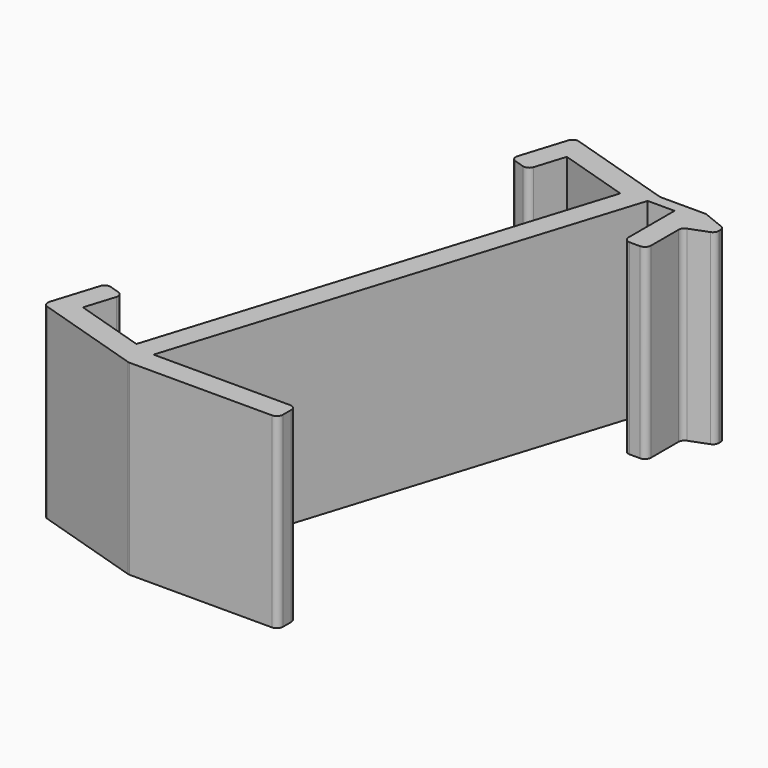
from build123d import *

# Parameters (mm, degrees)
F1_DEPTH = 25
F2_R     = 0.8


# Not quite as in the source:
# - a feature names something its author has since deleted; it is built from what else it names


with BuildPart() as f1:
    # F0 (on Top) → F1 (new body)
    with BuildSketch(Plane.XY):
        Polygon((-15.2705168036, 4.776119403), (-17.6585765051, -2.8591389988), (-14.7953546044, -3.7546613869), (-13.302817291, 1.0173751143), (-3.7587442887, -1.9676995126), (-21.9676995126, -60.1865448263), (-31.5117725148, -57.2014701994), (-30.0192352014, -52.4294336983), (-32.8824571021, -51.5339113102), (-35.2705168036, -59.169169712), (-20, -63.945289115), (-19.0616978853, -60.945289115), (-0.4691510573, -1.5), (3.1308489427, -1.5), (3.1308489427, -10), (6.1308489427, -10), (6.1308489427, -4.0311980993), (6.1308489427, 0), (0, 0), align=None)
        Polygon((0, -60.945289115), (-19.0616978853, -60.945289115), (-20, -63.945289115), (0, -63.945289115), align=None)
        Polygon((9.5918557882, -1.385692507), (6.1308489427, 0), (6.1308489427, -4.0311980993), (9.5918557882, -2.7201510966), align=None)
    extrude(amount=F1_DEPTH)

    # F2
    f2_edges = [f1.edges().sort_by_distance(p)[0] for p in [
        (-15.270517, 4.776119, 12.5),
        (-17.658577, -2.859139, 12.5),
        (-14.795355, -3.754661, 12.5),
        (-32.882457, -51.533911, 12.5),
        (-35.270517, -59.16917, 12.5),
        (-30.019235, -52.429434, 12.5),
        (-20, -63.945289, 12.5),
        (6.130849, -10, 12.5),
        (3.130849, -10, 12.5),
        (0, -60.945289, 12.5),
        (0, -63.945289, 12.5),
        (9.591856, -1.385693, 12.5),
        (9.591856, -2.720151, 12.5),
        (0, 0, 12.5),
        (6.130849, 0, 12.5),
        (6.130849, -4.031198, 12.5),
    ]]
    fillet(f2_edges, radius=F2_R)


solid = f1.part
